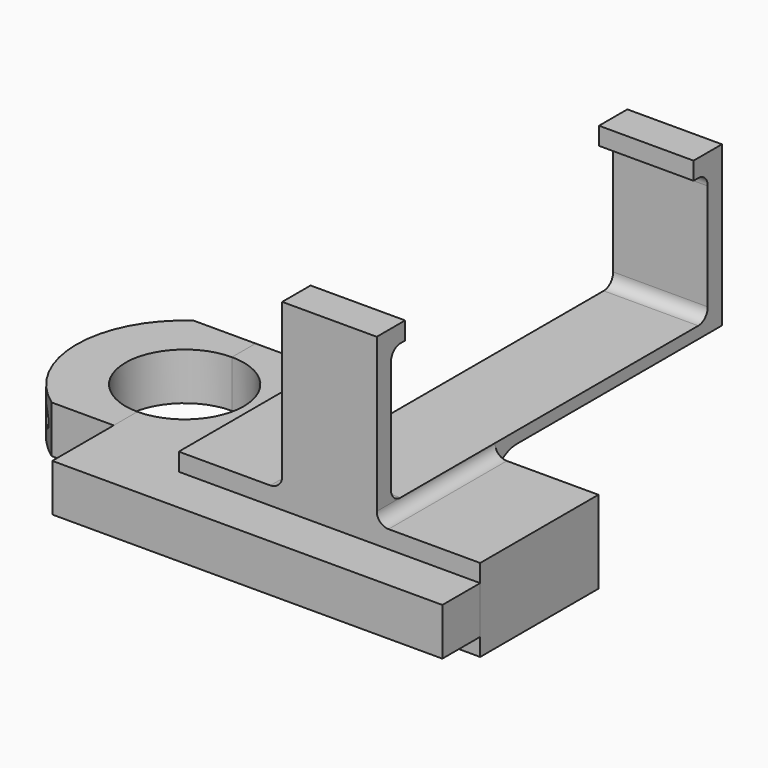
from build123d import *

# Parameters (mm, degrees)
F0_W         = 10.5
F0_H         = 5
F1_DEPTH     = 8
F2_R         = 1.5
F3_DEPTH     = 14.6382812683
F4_W         = 15
F4_H         = 5
F5_DEPTH     = 8
F6_R         = 1.5
F7_DEPTH     = 15
F8_W         = 51
F8_H         = 3
F8_H_2       = 8
F9_DEPTH     = 25
F11_DEPTH    = 22
F12_W        = 16
F12_H        = 48
F12_H_2      = 25
F13_DEPTH    = 2
F14_W        = 16
F14_H        = 3
F15_DEPTH    = 22
F16_W        = 16
F16_H        = 3
F17_DEPTH    = 3
F18_W        = 16
F18_H        = 3
F19_DEPTH    = 23
F20_W        = 16
F20_H        = 3
F21_DEPTH    = 3
F22_R        = 1.9999
F24_T1_DEPTH = 16


# Not quite as in the source:
# - a fillet or chamfer that OpenCascade refuses, or shapes differently, is made with other operations: its cross-section is extruded or revolved along the edge and cut away or added
# - two fillets or chamfers of one size are made in one step
# - a fillet or chamfer is up to 0.001 mm smaller than in the source, because OpenCascade refuses the exact size
# - a feature names something its author has since deleted; it is built from what else it names


with BuildPart() as f1:
    # F0 (on Top) → F1 (new body)
    with BuildSketch(Plane.XY):
        with Locations((-5.25, 12.5)):
            Rectangle(F0_W, F0_H)
        with BuildLine():
            ThreePointArc((0, -10), (-10, 0), (0, 10))
            Line((0, 10), (-10.5, 10))
            Line((-10.5, 10), (-10.5, 15))
            ThreePointArc((-10.5, 15), (-18.3098334236, 0), (-10.5, -15))
            Line((-10.5, -15), (-10.5, -10))
            Line((-10.5, -10), (0, -10))
        make_face()
        with Locations((-5.25, -12.5)):
            Rectangle(F0_W, F0_H)
    extrude(amount=F1_DEPTH)

    # F2 (on face) → F3 (cut, through all)
    with BuildSketch(Plane.YZ):
        with Locations((12.5, 4)):
            Circle(F2_R)
        with Locations((-12.5, 4)):
            Circle(F2_R)
    extrude(amount=-F3_DEPTH, mode=Mode.SUBTRACT)


with BuildPart() as f5:
    # F4 (on Top) → F5 (new body)
    with BuildSketch(Plane.XY):
        with BuildLine():
            Line((15, 10), (0, 10))
            ThreePointArc((0, 10), (10, 0), (0, -10))
            Line((0, -10), (15, -10))
            Line((15, -10), (15, 10))
        make_face()
        with Locations((7.5, 12.5)):
            Rectangle(F4_W, F4_H)
        with Locations((7.5, -12.5)):
            Rectangle(F4_W, F4_H)
        with Locations((7.5, -17.5)):
            Rectangle(F4_W, F4_H)
        Polygon((15, -20), (0, -20), (0, -28), (66, -28), (66, -20), align=None)
    extrude(amount=F5_DEPTH)

    # F6 (on face) → F7 (cut, through all)
    with BuildSketch(Plane.YZ.offset(15)):
        with Locations((-12.5, 4)):
            Circle(F6_R)
        with Locations((12.5, 4)):
            Circle(F6_R)
    extrude(amount=-F7_DEPTH, mode=Mode.SUBTRACT)


with BuildPart() as f9:
    # F8 (on face) → F9 (new body)
    with BuildSketch(Plane(origin=(0, -20, 0), x_dir=(-1, 0, 0), z_dir=(0, 1, 0))):
        with Locations((-40.5, 9.5)):
            Rectangle(F8_W, F8_H)
        with Locations((-40.5, 4)):
            Rectangle(F8_W, F8_H_2)
        with Locations((-40.5, -1.5)):
            Rectangle(F8_W, F8_H)
    extrude(amount=F9_DEPTH)

    # F10 (on face) → F11 (cut)
    with BuildSketch(Plane(origin=(0, 5, 0), x_dir=(-1, 0, 0), z_dir=(0, 1, 0))):
        with BuildLine():
            Line((-17.9999992251, 1.9999992251), (-17.9999992251, 6.0000007749))
            ThreePointArc((-17.9999992251, 6.0000007749), (-18.5857856628, 7.4142143372), (-19.9999992251, 8.0000007749))
            Line((-19.9999992251, 8.0000007749), (-61.0000007749, 8.0000007749))
            ThreePointArc((-61.0000007749, 8.0000007749), (-62.4142143372, 7.4142143372), (-63.0000007749, 6.0000007749))
            Line((-63.0000007749, 6.0000007749), (-63.0000007749, 1.9999992251))
            ThreePointArc((-63.0000007749, 1.9999992251), (-62.4142143372, 0.5857856628), (-61.0000007749, -7.749e-07))
            Line((-61.0000007749, -7.749e-07), (-19.9999992251, -7.749e-07))
            ThreePointArc((-19.9999992251, -7.749e-07), (-18.5857856628, 0.5857856628), (-17.9999992251, 1.9999992251))
        make_face()
    extrude(amount=-F11_DEPTH, mode=Mode.SUBTRACT)

    # F12 (on face) → F13 (join)
    with BuildSketch(Plane.XY.offset(11)):
        with Locations((40.5, 29)):
            Rectangle(F12_W, F12_H)
        with Locations((40.5, -7.5)):
            Rectangle(F12_W, F12_H_2)
    extrude(amount=F13_DEPTH)

    # F14 (on face) → F15 (join)
    with BuildSketch(Plane.XY.offset(13)):
        with Locations((40.5, 51.5)):
            Rectangle(F14_W, F14_H)
    extrude(amount=F15_DEPTH)

    # F16 (on face) → F17 (join)
    with BuildSketch(Plane.XY.offset(35)):
        with Locations((40.5, 48.5)):
            Rectangle(F16_W, F16_H)
        with Locations((40.5, 51.5)):
            Rectangle(F16_W, F16_H)
    extrude(amount=F17_DEPTH)

    # F18 (on face) → F19 (join)
    with BuildSketch(Plane.XY.offset(13)):
        with Locations((40.5, -18.5)):
            Rectangle(F18_W, F18_H)
    extrude(amount=F19_DEPTH)

    # F20 (on face) → F21 (join)
    with BuildSketch(Plane.XY.offset(36)):
        with Locations((40.5, -15.5)):
            Rectangle(F20_W, F20_H)
        with Locations((40.5, -18.5)):
            Rectangle(F20_W, F20_H)
    extrude(amount=F21_DEPTH)

    # F22 (radius 2 in the source; OpenCascade refuses exactly that, so slightly less here)
    f22_edges = [f9.edges().sort_by_distance(p)[0] for p in [
        (32.5, -7.5, 11),
        (48.5, -7.5, 11),
        (40.5, 50, 35),
        (40.5, 50, 13),
        (40.5, -17, 13),
        (40.5, -17, 36),
    ]]
    fillet(f22_edges, radius=F22_R)

    # F24: fillet of radius 5 on 1 edges, made by hand

    # F24_s2 → F24_t1 (join)
    with BuildSketch(Plane.YZ.offset(32.5)):
        with BuildLine():
            ThreePointArc((5, 8.0000007749), (6.8439629229, 10.1833003642), (9.5825753568, 11))
            Line((9.5825753568, 11), (5, 11))
            Line((5, 11), (5, 8.0000007749))
        make_face()
    extrude(amount=F24_T1_DEPTH)


solid = Compound([f1.part, f5.part, f9.part])
